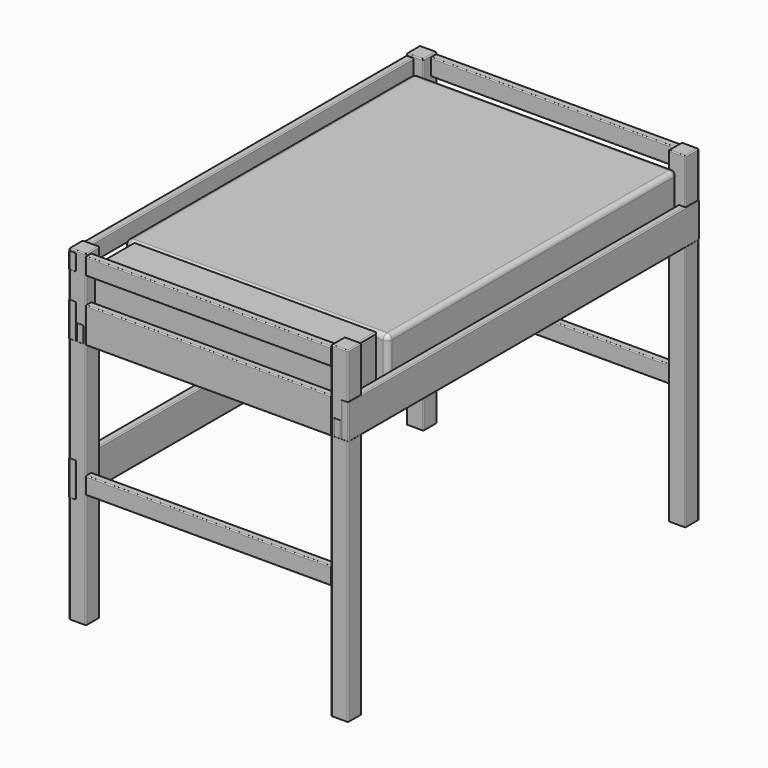
from build123d import *

# Parameters (mm, degrees)
F1_DEPTH       = 1700
F3_DEPTH       = 1141
F3_DEPTH_BACK  = 1141
F5_DEPTH       = 637.5
F5_DEPTH_BACK  = 637.5
F7_DEPTH       = 830
F7_DEPTH_BACK  = 1050
F8_W           = 260
F8_H           = 245
F9_DEPTH       = 630
F9_DEPTH_BACK  = 630
F8_H_2         = 12.5
F11_DEPTH      = 650
F11_DEPTH_BACK = 650
F12_R          = 5
F13_R          = 25
F14_R          = 5
F15_R          = 5
F15_2_R        = 5
F15_3_R        = 5
F15_4_R        = 5
F15_5_R        = 5
F15_6_R        = 5
F15_7_R        = 5
F15_8_R        = 5
F15_9_R        = 5
F15_10_R       = 5


# Not quite as in the source:
# - a feature names something its author has since deleted; it is built from what else it names


with BuildPart() as f1:
    # F0 (on Top) → F1 (new body)
    with BuildSketch(Plane.XY):
        with BuildLine():
            Line((-642.5, -1052.5), (-720, -1052.5))
            ThreePointArc((-720, -1052.5), (-723.5355339059, -1053.9644660941), (-725, -1057.5))
            Line((-725, -1057.5), (-725, -1135))
            ThreePointArc((-725, -1135), (-723.5355339059, -1138.5355339059), (-720, -1140))
            Line((-720, -1140), (-642.5, -1140))
            ThreePointArc((-642.5, -1140), (-638.9644660941, -1138.5355339059), (-637.5, -1135))
            Line((-637.5, -1135), (-637.5, -1057.5))
            ThreePointArc((-637.5, -1057.5), (-638.9644660941, -1053.9644660941), (-642.5, -1052.5))
        make_face()
    extrude(amount=F1_DEPTH)

    # F15#2
    f15_2_edges = [f1.edges().sort_by_distance(p)[0] for p in [
        (-637.5, -1096.25, 1700),
        (-638.964466, -1053.964466, 1700),
        (-681.25, -1052.5, 1700),
        (-723.535534, -1053.964466, 1700),
        (-725, -1096.25, 1700),
        (-723.535534, -1138.535534, 1700),
        (-681.25, -1140, 1700),
        (-638.964466, -1138.535534, 1700),
    ]]
    fillet(f15_2_edges, radius=F15_2_R)


with BuildPart() as f1b:
    # F0 (on Top) → F1, piece 2 (new body)
    with BuildSketch(Plane.XY):
        with BuildLine():
            Line((-642.5, 1140), (-720, 1140))
            ThreePointArc((-720, 1140), (-723.5355339059, 1138.5355339059), (-725, 1135))
            Line((-725, 1135), (-725, 1057.5))
            ThreePointArc((-725, 1057.5), (-723.5355339059, 1053.9644660941), (-720, 1052.5))
            Line((-720, 1052.5), (-642.5, 1052.5))
            ThreePointArc((-642.5, 1052.5), (-638.9644660941, 1053.9644660941), (-637.5, 1057.5))
            Line((-637.5, 1057.5), (-637.5, 1135))
            ThreePointArc((-637.5, 1135), (-638.9644660941, 1138.5355339059), (-642.5, 1140))
        make_face()
    extrude(amount=F1_DEPTH)

    # F15#9
    f15_9_edges = [f1b.edges().sort_by_distance(p)[0] for p in [
        (-638.964466, 1138.535534, 1700),
        (-681.25, 1140, 1700),
        (-723.535534, 1138.535534, 1700),
        (-725, 1096.25, 1700),
        (-723.535534, 1053.964466, 1700),
        (-681.25, 1052.5, 1700),
        (-638.964466, 1053.964466, 1700),
        (-637.5, 1096.25, 1700),
    ]]
    fillet(f15_9_edges, radius=F15_9_R)


with BuildPart() as f1c:
    # F0 (on Top) → F1, piece 3 (new body)
    with BuildSketch(Plane.XY):
        with BuildLine():
            Line((720, 1140), (642.5, 1140))
            ThreePointArc((642.5, 1140), (638.9644660941, 1138.5355339059), (637.5, 1135))
            Line((637.5, 1135), (637.5, 1057.5))
            ThreePointArc((637.5, 1057.5), (638.9644660941, 1053.9644660941), (642.5, 1052.5))
            Line((642.5, 1052.5), (720, 1052.5))
            ThreePointArc((720, 1052.5), (723.5355339059, 1053.9644660941), (725, 1057.5))
            Line((725, 1057.5), (725, 1135))
            ThreePointArc((725, 1135), (723.5355339059, 1138.5355339059), (720, 1140))
        make_face()
    extrude(amount=F1_DEPTH)

    # F15#8
    f15_8_edges = [f1c.edges().sort_by_distance(p)[0] for p in [
        (723.535534, 1138.535534, 1700),
        (681.25, 1140, 1700),
        (638.964466, 1138.535534, 1700),
        (637.5, 1096.25, 1700),
        (638.964466, 1053.964466, 1700),
        (681.25, 1052.5, 1700),
        (723.535534, 1053.964466, 1700),
        (725, 1096.25, 1700),
    ]]
    fillet(f15_8_edges, radius=F15_8_R)


with BuildPart() as f1d:
    # F0 (on Top) → F1, piece 4 (new body)
    with BuildSketch(Plane.XY):
        with BuildLine():
            Line((720, -1052.5), (642.5, -1052.5))
            ThreePointArc((642.5, -1052.5), (638.9644660941, -1053.9644660941), (637.5, -1057.5))
            Line((637.5, -1057.5), (637.5, -1135))
            ThreePointArc((637.5, -1135), (638.9644660941, -1138.5355339059), (642.5, -1140))
            Line((642.5, -1140), (720, -1140))
            ThreePointArc((720, -1140), (723.5355339059, -1138.5355339059), (725, -1135))
            Line((725, -1135), (725, -1057.5))
            ThreePointArc((725, -1057.5), (723.5355339059, -1053.9644660941), (720, -1052.5))
        make_face()
    extrude(amount=F1_DEPTH)

    # F15
    f15_edges = [f1d.edges().sort_by_distance(p)[0] for p in [
        (725, -1096.25, 1700),
        (723.535534, -1053.964466, 1700),
        (681.25, -1052.5, 1700),
        (638.964466, -1053.964466, 1700),
        (637.5, -1096.25, 1700),
        (638.964466, -1138.535534, 1700),
        (681.25, -1140, 1700),
        (723.535534, -1138.535534, 1700),
    ]]
    fillet(f15_edges, radius=F15_R)


with BuildPart() as f3:
    # F2 (on Front) → F3 (new body, two sides)
    with BuildSketch(Plane.XZ) as f3_sk:
        with BuildLine():
            Line((-694, 1466), (-722, 1466))
            ThreePointArc((-722, 1466), (-725.5355339059, 1464.5355339059), (-727, 1461))
            Line((-727, 1461), (-727, 1287))
            ThreePointArc((-727, 1287), (-725.5355339059, 1283.4644660941), (-722, 1282))
            Line((-722, 1282), (-694, 1282))
            ThreePointArc((-694, 1282), (-690.4644660941, 1283.4644660941), (-689, 1287))
            Line((-689, 1287), (-689, 1461))
            ThreePointArc((-689, 1461), (-690.4644660941, 1464.5355339059), (-694, 1466))
        make_face()
    extrude(amount=F3_DEPTH)
    extrude(f3_sk.sketch, amount=-F3_DEPTH_BACK)

    # F15#3
    f15_3_edges = [f3.edges().sort_by_distance(p)[0] for p in [
        (-690.464466, -1141, 1464.535534),
        (-708, -1141, 1466),
        (-725.535534, -1141, 1464.535534),
        (-727, -1141, 1374),
        (-725.535534, -1141, 1283.464466),
        (-708, -1141, 1282),
        (-690.464466, -1141, 1283.464466),
        (-689, -1141, 1374),
        (-690.464466, 1141, 1464.535534),
        (-708, 1141, 1466),
        (-725.535534, 1141, 1464.535534),
        (-727, 1141, 1374),
        (-725.535534, 1141, 1283.464466),
        (-708, 1141, 1282),
        (-690.464466, 1141, 1283.464466),
        (-689, 1141, 1374),
    ]]
    fillet(f15_3_edges, radius=F15_3_R)


with BuildPart() as f3b:
    # F2 (on Front) → F3, piece 2 (new body, two sides)
    with BuildSketch(Plane.XZ) as f3_2_sk:
        with BuildLine():
            ThreePointArc((727, 1461), (725.5355339059, 1464.5355339059), (722, 1466))
            Line((722, 1466), (694, 1466))
            ThreePointArc((694, 1466), (690.4644660941, 1464.5355339059), (689, 1461))
            Line((689, 1461), (689, 1287))
            ThreePointArc((689, 1287), (690.4644660941, 1283.4644660941), (694, 1282))
            Line((694, 1282), (722, 1282))
            ThreePointArc((722, 1282), (725.5355339059, 1283.4644660941), (727, 1287))
            Line((727, 1287), (727, 1461))
        make_face()
    extrude(amount=F3_DEPTH)
    extrude(f3_2_sk.sketch, amount=-F3_DEPTH_BACK)

    # F15#5
    f15_5_edges = [f3b.edges().sort_by_distance(p)[0] for p in [
        (725.535534, -1141, 1464.535534),
        (708, -1141, 1466),
        (690.464466, -1141, 1464.535534),
        (689, -1141, 1374),
        (690.464466, -1141, 1283.464466),
        (708, -1141, 1282),
        (725.535534, -1141, 1283.464466),
        (727, -1141, 1374),
        (725.535534, 1141, 1464.535534),
        (708, 1141, 1466),
        (690.464466, 1141, 1464.535534),
        (689, 1141, 1374),
        (690.464466, 1141, 1283.464466),
        (708, 1141, 1282),
        (725.535534, 1141, 1283.464466),
        (727, 1141, 1374),
    ]]
    fillet(f15_5_edges, radius=F15_5_R)


with BuildPart() as f3c:
    # F2 (on Front) → F3, piece 3 (new body, two sides)
    with BuildSketch(Plane.XZ) as f3_3_sk:
        with BuildLine():
            Line((-694, 740), (-722, 740))
            ThreePointArc((-722, 740), (-725.5355339059, 738.5355339059), (-727, 735))
            Line((-727, 735), (-727, 561))
            ThreePointArc((-727, 561), (-725.5355339059, 557.4644660941), (-722, 556))
            Line((-722, 556), (-694, 556))
            ThreePointArc((-694, 556), (-690.4644660941, 557.4644660941), (-689, 561))
            Line((-689, 561), (-689, 735))
            ThreePointArc((-689, 735), (-690.4644660941, 738.5355339059), (-694, 740))
        make_face()
    extrude(amount=F3_DEPTH)
    extrude(f3_3_sk.sketch, amount=-F3_DEPTH_BACK)

    # F15#7
    f15_7_edges = [f3c.edges().sort_by_distance(p)[0] for p in [
        (-690.464466, -1141, 738.535534),
        (-708, -1141, 740),
        (-725.535534, -1141, 738.535534),
        (-727, -1141, 648),
        (-725.535534, -1141, 557.464466),
        (-708, -1141, 556),
        (-690.464466, -1141, 557.464466),
        (-689, -1141, 648),
        (-690.464466, 1141, 738.535534),
        (-708, 1141, 740),
        (-725.535534, 1141, 738.535534),
        (-727, 1141, 648),
        (-725.535534, 1141, 557.464466),
        (-708, 1141, 556),
        (-690.464466, 1141, 557.464466),
        (-689, 1141, 648),
    ]]
    fillet(f15_7_edges, radius=F15_7_R)


with BuildPart() as f3d:
    # F2 (on Front) → F3, piece 4 (new body, two sides)
    with BuildSketch(Plane.XZ) as f3_4_sk:
        with BuildLine():
            ThreePointArc((-650, 1366), (-651.4644660941, 1369.5355339059), (-655, 1371))
            Line((-655, 1371), (-683, 1371))
            ThreePointArc((-683, 1371), (-686.5355339059, 1369.5355339059), (-688, 1366))
            Line((-688, 1366), (-688, 1287))
            ThreePointArc((-688, 1287), (-686.5355339059, 1283.4644660941), (-683, 1282))
            Line((-683, 1282), (-655, 1282))
            ThreePointArc((-655, 1282), (-651.4644660941, 1283.4644660941), (-650, 1287))
            Line((-650, 1287), (-650, 1366))
        make_face()
    extrude(amount=F3_DEPTH)
    extrude(f3_4_sk.sketch, amount=-F3_DEPTH_BACK)

    # F15#4
    f15_4_edges = [f3d.edges().sort_by_distance(p)[0] for p in [
        (-651.464466, -1141, 1369.535534),
        (-669, -1141, 1371),
        (-686.535534, -1141, 1369.535534),
        (-688, -1141, 1326.5),
        (-686.535534, -1141, 1283.464466),
        (-669, -1141, 1282),
        (-651.464466, -1141, 1283.464466),
        (-650, -1141, 1326.5),
        (-651.464466, 1141, 1369.535534),
        (-669, 1141, 1371),
        (-686.535534, 1141, 1369.535534),
        (-688, 1141, 1326.5),
        (-686.535534, 1141, 1283.464466),
        (-669, 1141, 1282),
        (-651.464466, 1141, 1283.464466),
        (-650, 1141, 1326.5),
    ]]
    fillet(f15_4_edges, radius=F15_4_R)


with BuildPart() as f3e:
    # F2 (on Front) → F3, piece 5 (new body, two sides)
    with BuildSketch(Plane.XZ) as f3_5_sk:
        with BuildLine():
            Line((683, 1371), (655, 1371))
            ThreePointArc((655, 1371), (651.4644660941, 1369.5355339059), (650, 1366))
            Line((650, 1366), (650, 1287))
            ThreePointArc((650, 1287), (651.4644660941, 1283.4644660941), (655, 1282))
            Line((655, 1282), (683, 1282))
            ThreePointArc((683, 1282), (686.5355339059, 1283.4644660941), (688, 1287))
            Line((688, 1287), (688, 1366))
            ThreePointArc((688, 1366), (686.5355339059, 1369.5355339059), (683, 1371))
        make_face()
    extrude(amount=F3_DEPTH)
    extrude(f3_5_sk.sketch, amount=-F3_DEPTH_BACK)

    # F15#6
    f15_6_edges = [f3e.edges().sort_by_distance(p)[0] for p in [
        (686.535534, -1141, 1369.535534),
        (669, -1141, 1371),
        (651.464466, -1141, 1369.535534),
        (650, -1141, 1326.5),
        (651.464466, -1141, 1283.464466),
        (669, -1141, 1282),
        (686.535534, -1141, 1283.464466),
        (688, -1141, 1326.5),
        (686.535534, 1141, 1369.535534),
        (669, 1141, 1371),
        (651.464466, 1141, 1369.535534),
        (650, 1141, 1326.5),
        (651.464466, 1141, 1283.464466),
        (669, 1141, 1282),
        (686.535534, 1141, 1283.464466),
        (688, 1141, 1326.5),
    ]]
    fillet(f15_6_edges, radius=F15_6_R)


with BuildPart() as f3f:
    # F2 (on Front) → F3, piece 6 (new body, two sides)
    with BuildSketch(Plane.XZ) as f3_6_sk:
        with BuildLine():
            Line((-694, 1689), (-722, 1689))
            ThreePointArc((-722, 1689), (-725.5355339059, 1687.5355339059), (-727, 1684))
            Line((-727, 1684), (-727, 1605))
            ThreePointArc((-727, 1605), (-725.5355339059, 1601.4644660941), (-722, 1600))
            Line((-722, 1600), (-694, 1600))
            ThreePointArc((-694, 1600), (-690.4644660941, 1601.4644660941), (-689, 1605))
            Line((-689, 1605), (-689, 1684))
            ThreePointArc((-689, 1684), (-690.4644660941, 1687.5355339059), (-694, 1689))
        make_face()
    extrude(amount=F3_DEPTH)
    extrude(f3_6_sk.sketch, amount=-F3_DEPTH_BACK)

    # F15#10
    f15_10_edges = [f3f.edges().sort_by_distance(p)[0] for p in [
        (-690.464466, -1141, 1687.535534),
        (-708, -1141, 1689),
        (-725.535534, -1141, 1687.535534),
        (-727, -1141, 1644.5),
        (-725.535534, -1141, 1601.464466),
        (-708, -1141, 1600),
        (-690.464466, -1141, 1601.464466),
        (-689, -1141, 1644.5),
        (-690.464466, 1141, 1687.535534),
        (-708, 1141, 1689),
        (-725.535534, 1141, 1687.535534),
        (-727, 1141, 1644.5),
        (-725.535534, 1141, 1601.464466),
        (-708, 1141, 1600),
        (-690.464466, 1141, 1601.464466),
        (-689, 1141, 1644.5),
    ]]
    fillet(f15_10_edges, radius=F15_10_R)


with BuildPart() as f5:
    # F4 (on Right) → F5 (new body, two sides)
    with BuildSketch(Plane.YZ) as f5_sk:
        with BuildLine():
            Line((-1108, 1689), (-1136, 1689))
            ThreePointArc((-1136, 1689), (-1139.5355339059, 1687.5355339059), (-1141, 1684))
            Line((-1141, 1684), (-1141, 1605))
            ThreePointArc((-1141, 1605), (-1139.5355339059, 1601.4644660941), (-1136, 1600))
            Line((-1136, 1600), (-1108, 1600))
            ThreePointArc((-1108, 1600), (-1104.4644660941, 1601.4644660941), (-1103, 1605))
            Line((-1103, 1605), (-1103, 1684))
            ThreePointArc((-1103, 1684), (-1104.4644660941, 1687.5355339059), (-1108, 1689))
        make_face()
    extrude(amount=F5_DEPTH)
    extrude(f5_sk.sketch, amount=-F5_DEPTH_BACK)


with BuildPart() as f5b:
    # F4 (on Right) → F5, piece 2 (new body, two sides)
    with BuildSketch(Plane.YZ) as f5_2_sk:
        with BuildLine():
            ThreePointArc((1141, 1684), (1139.5355339059, 1687.5355339059), (1136, 1689))
            Line((1136, 1689), (1108, 1689))
            ThreePointArc((1108, 1689), (1104.4644660941, 1687.5355339059), (1103, 1684))
            Line((1103, 1684), (1103, 1605))
            ThreePointArc((1103, 1605), (1104.4644660941, 1601.4644660941), (1108, 1600))
            Line((1108, 1600), (1136, 1600))
            ThreePointArc((1136, 1600), (1139.5355339059, 1601.4644660941), (1141, 1605))
            Line((1141, 1605), (1141, 1684))
        make_face()
    extrude(amount=F5_DEPTH)
    extrude(f5_2_sk.sketch, amount=-F5_DEPTH_BACK)


with BuildPart() as f5c:
    # F4 (on Right) → F5, piece 3 (new body, two sides)
    with BuildSketch(Plane.YZ) as f5_3_sk:
        with BuildLine():
            Line((-1108, 1466), (-1136, 1466))
            ThreePointArc((-1136, 1466), (-1139.5355339059, 1464.5355339059), (-1141, 1461))
            Line((-1141, 1461), (-1141, 1287.1))
            ThreePointArc((-1141, 1287.1), (-1139.5062445841, 1283.4937554159), (-1135.9, 1282))
            Line((-1135.9, 1282), (-1108, 1282))
            ThreePointArc((-1108, 1282), (-1104.4644660941, 1283.4644660941), (-1103, 1287))
            Line((-1103, 1287), (-1103, 1461))
            ThreePointArc((-1103, 1461), (-1104.4644660941, 1464.5355339059), (-1108, 1466))
        make_face()
    extrude(amount=F5_DEPTH)
    extrude(f5_3_sk.sketch, amount=-F5_DEPTH_BACK)


with BuildPart() as f5d:
    # F4 (on Right) → F5, piece 4 (new body, two sides)
    with BuildSketch(Plane.YZ) as f5_4_sk:
        with BuildLine():
            ThreePointArc((1141, 1461), (1139.5355339059, 1464.5355339059), (1136, 1466))
            Line((1136, 1466), (1108, 1466))
            ThreePointArc((1108, 1466), (1104.4644660941, 1464.5355339059), (1103, 1461))
            Line((1103, 1461), (1103, 1287))
            ThreePointArc((1103, 1287), (1104.4644660941, 1283.4644660941), (1108, 1282))
            Line((1108, 1282), (1136, 1282))
            ThreePointArc((1136, 1282), (1139.5355339059, 1283.4644660941), (1141, 1287))
            Line((1141, 1287), (1141, 1461))
        make_face()
    extrude(amount=F5_DEPTH)
    extrude(f5_4_sk.sketch, amount=-F5_DEPTH_BACK)


with BuildPart() as f5e:
    # F4 (on Right) → F5, piece 5 (new body, two sides)
    with BuildSketch(Plane.YZ) as f5_5_sk:
        with BuildLine():
            Line((-1108, 685), (-1136, 685))
            ThreePointArc((-1136, 685), (-1139.5355339059, 683.5355339059), (-1141, 680))
            Line((-1141, 680), (-1141, 601))
            ThreePointArc((-1141, 601), (-1139.5355339059, 597.4644660941), (-1136, 596))
            Line((-1136, 596), (-1108, 596))
            ThreePointArc((-1108, 596), (-1104.4644660941, 597.4644660941), (-1103, 601))
            Line((-1103, 601), (-1103, 680))
            ThreePointArc((-1103, 680), (-1104.4644660941, 683.5355339059), (-1108, 685))
        make_face()
    extrude(amount=F5_DEPTH)
    extrude(f5_5_sk.sketch, amount=-F5_DEPTH_BACK)


with BuildPart() as f5f:
    # F4 (on Right) → F5, piece 6 (new body, two sides)
    with BuildSketch(Plane.YZ) as f5_6_sk:
        with BuildLine():
            Line((1108, 596), (1136, 596))
            ThreePointArc((1136, 596), (1139.5355339059, 597.4644660941), (1141, 601))
            Line((1141, 601), (1141, 680))
            ThreePointArc((1141, 680), (1139.5355339059, 683.5355339059), (1136, 685))
            Line((1136, 685), (1108, 685))
            ThreePointArc((1108, 685), (1104.4644660941, 683.5355339059), (1103, 680))
            Line((1103, 680), (1103, 601))
            ThreePointArc((1103, 601), (1104.4644660941, 597.4644660941), (1108, 596))
        make_face()
    extrude(amount=F5_DEPTH)
    extrude(f5_6_sk.sketch, amount=-F5_DEPTH_BACK)


with BuildPart() as f7:
    # F6 (on Front) → F7 (new body, two sides)
    with BuildSketch(Plane.XZ) as f7_sk:
        with BuildLine():
            Line((660, 1626), (-660, 1626))
            ThreePointArc((-660, 1626), (-677.6776695297, 1618.6776695297), (-685, 1601))
            Line((-685, 1601), (-685, 1397))
            ThreePointArc((-685, 1397), (-677.6776695297, 1379.3223304703), (-660, 1372))
            Line((-660, 1372), (660, 1372))
            ThreePointArc((660, 1372), (677.6776695297, 1379.3223304703), (685, 1397))
            Line((685, 1397), (685, 1601))
            ThreePointArc((685, 1601), (677.6776695297, 1618.6776695297), (660, 1626))
        make_face()
    extrude(amount=F7_DEPTH)
    extrude(f7_sk.sketch, amount=-F7_DEPTH_BACK)

    # F13
    f13_edges = [f7.edges().sort_by_distance(p)[0] for p in [
        (685, -830, 1499),
        (677.67767, -830, 1618.67767),
        (0, -830, 1626),
        (-677.67767, -830, 1618.67767),
        (-685, -830, 1499),
        (-677.67767, -830, 1379.32233),
        (0, -830, 1372),
        (677.67767, -830, 1379.32233),
        (685, 1050, 1499),
        (677.67767, 1050, 1618.67767),
        (0, 1050, 1626),
        (-677.67767, 1050, 1618.67767),
        (-685, 1050, 1499),
        (-677.67767, 1050, 1379.32233),
        (0, 1050, 1372),
        (677.67767, 1050, 1379.32233),
    ]]
    fillet(f13_edges, radius=F13_R)


with BuildPart() as f9:
    # F8 (on Right) → F9 (new body, two sides)
    with BuildSketch(Plane.YZ) as f9_sk:
        with Locations((-965, 1494.5)):
            Rectangle(F8_W, F8_H)
    extrude(amount=F9_DEPTH)
    extrude(f9_sk.sketch, amount=-F9_DEPTH_BACK)

    # F14
    f14_edges = [f9.edges().sort_by_distance(p)[0] for p in [
        (-630, -835, 1494.5),
        (-630, -965, 1617),
        (-630, -1095, 1494.5),
        (-630, -965, 1372),
        (630, -835, 1494.5),
        (630, -965, 1617),
        (630, -1095, 1494.5),
        (630, -965, 1372),
        (0, -1095, 1372),
        (0, -1095, 1617),
        (0, -835, 1372),
        (0, -835, 1617),
    ]]
    fillet(f14_edges, radius=F14_R)


with BuildPart() as f9b:
    # F8 (on Right) → F9, piece 2 (new body, two sides)
    with BuildSketch(Plane.YZ) as f9_2_sk:
        with Locations((-965, 1625.75)):
            Rectangle(F8_W, F8_H_2)
    extrude(amount=F9_DEPTH)
    extrude(f9_2_sk.sketch, amount=-F9_DEPTH_BACK)

    # F12
    f12_edges = [f9b.edges().sort_by_distance(p)[0] for p in [
        (0, -835, 1632),
        (630, -965, 1632),
        (0, -1095, 1632),
        (-630, -965, 1632),
        (630, -965, 1619.5),
        (0, -835, 1619.5),
        (-630, -965, 1619.5),
        (0, -1095, 1619.5),
        (630, -1095, 1625.75),
        (630, -835, 1625.75),
        (-630, -1095, 1625.75),
        (-630, -835, 1625.75),
    ]]
    fillet(f12_edges, radius=F12_R)


with BuildPart() as f11:
    # F10 (on Right) → F11 (new body, two sides)
    with BuildSketch(Plane.YZ) as f11_sk:
        with BuildLine():
            Line((-966, 1370), (-1045, 1370))
            ThreePointArc((-1045, 1370), (-1048.5355339059, 1368.5355339059), (-1050, 1365))
            Line((-1050, 1365), (-1050, 1337))
            ThreePointArc((-1050, 1337), (-1048.5355339059, 1333.4644660941), (-1045, 1332))
            Line((-1045, 1332), (-966, 1332))
            ThreePointArc((-966, 1332), (-962.4644660941, 1333.4644660941), (-961, 1337))
            Line((-961, 1337), (-961, 1365))
            ThreePointArc((-961, 1365), (-962.4644660941, 1368.5355339059), (-966, 1370))
        make_face()
    extrude(amount=F11_DEPTH)
    extrude(f11_sk.sketch, amount=-F11_DEPTH_BACK)


with BuildPart() as f11b:
    # F10 (on Right) → F11, piece 2 (new body, two sides)
    with BuildSketch(Plane.YZ) as f11_2_sk:
        with BuildLine():
            Line((-798.25, 1370), (-877.25, 1370))
            ThreePointArc((-877.25, 1370), (-880.7855339059, 1368.5355339059), (-882.25, 1365))
            Line((-882.25, 1365), (-882.25, 1337))
            ThreePointArc((-882.25, 1337), (-880.7855339059, 1333.4644660941), (-877.25, 1332))
            Line((-877.25, 1332), (-798.25, 1332))
            ThreePointArc((-798.25, 1332), (-794.7144660941, 1333.4644660941), (-793.25, 1337))
            Line((-793.25, 1337), (-793.25, 1365))
            ThreePointArc((-793.25, 1365), (-794.7144660941, 1368.5355339059), (-798.25, 1370))
        make_face()
    extrude(amount=F11_DEPTH)
    extrude(f11_2_sk.sketch, amount=-F11_DEPTH_BACK)


with BuildPart() as f11c:
    # F10 (on Right) → F11, piece 3 (new body, two sides)
    with BuildSketch(Plane.YZ) as f11_3_sk:
        with BuildLine():
            Line((-630.5, 1370), (-709.5, 1370))
            ThreePointArc((-709.5, 1370), (-713.0355339059, 1368.5355339059), (-714.5, 1365))
            Line((-714.5, 1365), (-714.5, 1337))
            ThreePointArc((-714.5, 1337), (-713.0355339059, 1333.4644660941), (-709.5, 1332))
            Line((-709.5, 1332), (-630.5, 1332))
            ThreePointArc((-630.5, 1332), (-626.9644660941, 1333.4644660941), (-625.5, 1337))
            Line((-625.5, 1337), (-625.5, 1365))
            ThreePointArc((-625.5, 1365), (-626.9644660941, 1368.5355339059), (-630.5, 1370))
        make_face()
    extrude(amount=F11_DEPTH)
    extrude(f11_3_sk.sketch, amount=-F11_DEPTH_BACK)


with BuildPart() as f11d:
    # F10 (on Right) → F11, piece 4 (new body, two sides)
    with BuildSketch(Plane.YZ) as f11_4_sk:
        with BuildLine():
            Line((-462.75, 1370), (-541.75, 1370))
            ThreePointArc((-541.75, 1370), (-545.2855339059, 1368.5355339059), (-546.75, 1365))
            Line((-546.75, 1365), (-546.75, 1337))
            ThreePointArc((-546.75, 1337), (-545.2855339059, 1333.4644660941), (-541.75, 1332))
            Line((-541.75, 1332), (-462.75, 1332))
            ThreePointArc((-462.75, 1332), (-459.2144660941, 1333.4644660941), (-457.75, 1337))
            Line((-457.75, 1337), (-457.75, 1365))
            ThreePointArc((-457.75, 1365), (-459.2144660941, 1368.5355339059), (-462.75, 1370))
        make_face()
    extrude(amount=F11_DEPTH)
    extrude(f11_4_sk.sketch, amount=-F11_DEPTH_BACK)


with BuildPart() as f11e:
    # F10 (on Right) → F11, piece 5 (new body, two sides)
    with BuildSketch(Plane.YZ) as f11_5_sk:
        with BuildLine():
            Line((-295, 1370), (-374, 1370))
            ThreePointArc((-374, 1370), (-377.5355339059, 1368.5355339059), (-379, 1365))
            Line((-379, 1365), (-379, 1337))
            ThreePointArc((-379, 1337), (-377.5355339059, 1333.4644660941), (-374, 1332))
            Line((-374, 1332), (-295, 1332))
            ThreePointArc((-295, 1332), (-291.4644660941, 1333.4644660941), (-290, 1337))
            Line((-290, 1337), (-290, 1365))
            ThreePointArc((-290, 1365), (-291.4644660941, 1368.5355339059), (-295, 1370))
        make_face()
    extrude(amount=F11_DEPTH)
    extrude(f11_5_sk.sketch, amount=-F11_DEPTH_BACK)


with BuildPart() as f11f:
    # F10 (on Right) → F11, piece 6 (new body, two sides)
    with BuildSketch(Plane.YZ) as f11_6_sk:
        with BuildLine():
            Line((-127.25, 1370), (-206.25, 1370))
            ThreePointArc((-206.25, 1370), (-209.7855339059, 1368.5355339059), (-211.25, 1365))
            Line((-211.25, 1365), (-211.25, 1337))
            ThreePointArc((-211.25, 1337), (-209.7855339059, 1333.4644660941), (-206.25, 1332))
            Line((-206.25, 1332), (-127.25, 1332))
            ThreePointArc((-127.25, 1332), (-123.7144660941, 1333.4644660941), (-122.25, 1337))
            Line((-122.25, 1337), (-122.25, 1365))
            ThreePointArc((-122.25, 1365), (-123.7144660941, 1368.5355339059), (-127.25, 1370))
        make_face()
    extrude(amount=F11_DEPTH)
    extrude(f11_6_sk.sketch, amount=-F11_DEPTH_BACK)


with BuildPart() as f11g:
    # F10 (on Right) → F11, piece 7 (new body, two sides)
    with BuildSketch(Plane.YZ) as f11_7_sk:
        with BuildLine():
            Line((40.5, 1370), (-38.5, 1370))
            ThreePointArc((-38.5, 1370), (-42.0355339059, 1368.5355339059), (-43.5, 1365))
            Line((-43.5, 1365), (-43.5, 1337))
            ThreePointArc((-43.5, 1337), (-42.0355339059, 1333.4644660941), (-38.5, 1332))
            Line((-38.5, 1332), (40.5, 1332))
            ThreePointArc((40.5, 1332), (44.0355339059, 1333.4644660941), (45.5, 1337))
            Line((45.5, 1337), (45.5, 1365))
            ThreePointArc((45.5, 1365), (44.0355339059, 1368.5355339059), (40.5, 1370))
        make_face()
    extrude(amount=F11_DEPTH)
    extrude(f11_7_sk.sketch, amount=-F11_DEPTH_BACK)


with BuildPart() as f11h:
    # F10 (on Right) → F11, piece 8 (new body, two sides)
    with BuildSketch(Plane.YZ) as f11_8_sk:
        with BuildLine():
            Line((208.25, 1370), (129.25, 1370))
            ThreePointArc((129.25, 1370), (125.7144660941, 1368.5355339059), (124.25, 1365))
            Line((124.25, 1365), (124.25, 1337))
            ThreePointArc((124.25, 1337), (125.7144660941, 1333.4644660941), (129.25, 1332))
            Line((129.25, 1332), (208.25, 1332))
            ThreePointArc((208.25, 1332), (211.7855339059, 1333.4644660941), (213.25, 1337))
            Line((213.25, 1337), (213.25, 1365))
            ThreePointArc((213.25, 1365), (211.7855339059, 1368.5355339059), (208.25, 1370))
        make_face()
    extrude(amount=F11_DEPTH)
    extrude(f11_8_sk.sketch, amount=-F11_DEPTH_BACK)


with BuildPart() as f11i:
    # F10 (on Right) → F11, piece 9 (new body, two sides)
    with BuildSketch(Plane.YZ) as f11_9_sk:
        with BuildLine():
            Line((376, 1370), (297, 1370))
            ThreePointArc((297, 1370), (293.4644660941, 1368.5355339059), (292, 1365))
            Line((292, 1365), (292, 1337))
            ThreePointArc((292, 1337), (293.4644660941, 1333.4644660941), (297, 1332))
            Line((297, 1332), (376, 1332))
            ThreePointArc((376, 1332), (379.5355339059, 1333.4644660941), (381, 1337))
            Line((381, 1337), (381, 1365))
            ThreePointArc((381, 1365), (379.5355339059, 1368.5355339059), (376, 1370))
        make_face()
    extrude(amount=F11_DEPTH)
    extrude(f11_9_sk.sketch, amount=-F11_DEPTH_BACK)


with BuildPart() as f11j:
    # F10 (on Right) → F11, piece 10 (new body, two sides)
    with BuildSketch(Plane.YZ) as f11_10_sk:
        with BuildLine():
            Line((543.75, 1370), (464.75, 1370))
            ThreePointArc((464.75, 1370), (461.2144660941, 1368.5355339059), (459.75, 1365))
            Line((459.75, 1365), (459.75, 1337))
            ThreePointArc((459.75, 1337), (461.2144660941, 1333.4644660941), (464.75, 1332))
            Line((464.75, 1332), (543.75, 1332))
            ThreePointArc((543.75, 1332), (547.2855339059, 1333.4644660941), (548.75, 1337))
            Line((548.75, 1337), (548.75, 1365))
            ThreePointArc((548.75, 1365), (547.2855339059, 1368.5355339059), (543.75, 1370))
        make_face()
    extrude(amount=F11_DEPTH)
    extrude(f11_10_sk.sketch, amount=-F11_DEPTH_BACK)


with BuildPart() as f11k:
    # F10 (on Right) → F11, piece 11 (new body, two sides)
    with BuildSketch(Plane.YZ) as f11_11_sk:
        with BuildLine():
            Line((711.5, 1370), (632.5, 1370))
            ThreePointArc((632.5, 1370), (628.9644660941, 1368.5355339059), (627.5, 1365))
            Line((627.5, 1365), (627.5, 1337))
            ThreePointArc((627.5, 1337), (628.9644660941, 1333.4644660941), (632.5, 1332))
            Line((632.5, 1332), (711.5, 1332))
            ThreePointArc((711.5, 1332), (715.0355339059, 1333.4644660941), (716.5, 1337))
            Line((716.5, 1337), (716.5, 1365))
            ThreePointArc((716.5, 1365), (715.0355339059, 1368.5355339059), (711.5, 1370))
        make_face()
    extrude(amount=F11_DEPTH)
    extrude(f11_11_sk.sketch, amount=-F11_DEPTH_BACK)


with BuildPart() as f11l:
    # F10 (on Right) → F11, piece 12 (new body, two sides)
    with BuildSketch(Plane.YZ) as f11_12_sk:
        with BuildLine():
            Line((879.25, 1370), (800.25, 1370))
            ThreePointArc((800.25, 1370), (796.7144660941, 1368.5355339059), (795.25, 1365))
            Line((795.25, 1365), (795.25, 1337))
            ThreePointArc((795.25, 1337), (796.7144660941, 1333.4644660941), (800.25, 1332))
            Line((800.25, 1332), (879.25, 1332))
            ThreePointArc((879.25, 1332), (882.7855339059, 1333.4644660941), (884.25, 1337))
            Line((884.25, 1337), (884.25, 1365))
            ThreePointArc((884.25, 1365), (882.7855339059, 1368.5355339059), (879.25, 1370))
        make_face()
    extrude(amount=F11_DEPTH)
    extrude(f11_12_sk.sketch, amount=-F11_DEPTH_BACK)


with BuildPart() as f11m:
    # F10 (on Right) → F11, piece 13 (new body, two sides)
    with BuildSketch(Plane.YZ) as f11_13_sk:
        with BuildLine():
            Line((1047, 1370), (968, 1370))
            ThreePointArc((968, 1370), (964.4644660941, 1368.5355339059), (963, 1365))
            Line((963, 1365), (963, 1337))
            ThreePointArc((963, 1337), (964.4644660941, 1333.4644660941), (968, 1332))
            Line((968, 1332), (1047, 1332))
            ThreePointArc((1047, 1332), (1050.5355339059, 1333.4644660941), (1052, 1337))
            Line((1052, 1337), (1052, 1365))
            ThreePointArc((1052, 1365), (1050.5355339059, 1368.5355339059), (1047, 1370))
        make_face()
    extrude(amount=F11_DEPTH)
    extrude(f11_13_sk.sketch, amount=-F11_DEPTH_BACK)


solid = Compound([f1.part, f1b.part, f1c.part, f1d.part, f3.part, f3b.part, f3c.part, f3d.part, f3e.part, f3f.part, f5.part, f5b.part, f5c.part, f5d.part, f5e.part, f5f.part, f7.part, f9.part, f9b.part, f11.part, f11b.part, f11c.part, f11d.part, f11e.part, f11f.part, f11g.part, f11h.part, f11i.part, f11j.part, f11k.part, f11l.part, f11m.part])
